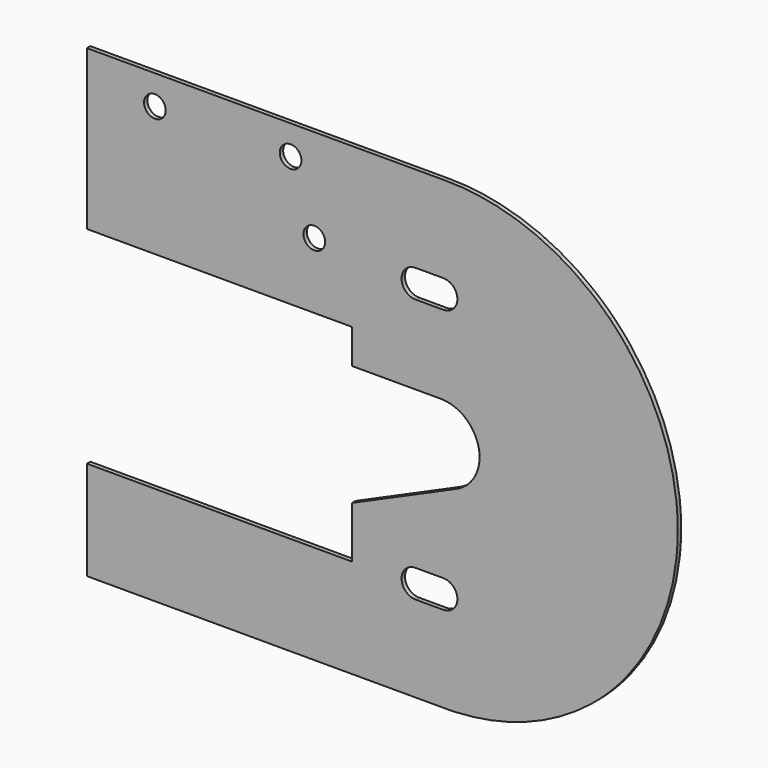
from build123d import *

# Parameters (mm, degrees)
F0_R     = 4.0005
F1_DEPTH = 1.5748


with BuildPart() as f1:
    # F0 (on Front) → F1 (new body)
    with BuildSketch(Plane.XZ):
        with BuildLine():
            Line((732.4313869209, 36.5125), (732.4313869209, 0))
            Line((732.4313869209, 0), (864.6383869209, 0))
            ThreePointArc((864.6383869209, 0), (866.7557920134, 0.0261539128), (868.8719051041, 0.1045996926))
            ThreePointArc((868.8719051041, 0.1045996926), (878.3590689291, 1.1051529768), (887.6763155537, 3.1536401389))
            ThreePointArc((887.6763155537, 3.1536401389), (903.696677756, 9.4149381337), (918.1445842563, 18.748418483))
            ThreePointArc((918.1445842563, 18.748418483), (921.7883869209, 21.8293575429), (925.2551157381, 25.1082711828))
            Line((925.2551157381, 25.1082711828), (873.8802209099, 76.483166011))
            ThreePointArc((873.8802209099, 76.483166011), (871.5444569052, 74.2857554291), (868.7774235028, 72.664665394))
            Line((868.7774235028, 72.664665394), (830.2213869209, 55.5625))
            Line((830.2213869209, 55.5625), (830.2213869209, 36.5125))
            Line((830.2213869209, 36.5125), (747.6713869209, 36.5125))
            Line((747.6713869209, 36.5125), (732.4313869209, 36.5125))
        make_face()
        with BuildLine():
            ThreePointArc((853.6528869209, 31.8135), (848.5093869209, 36.957), (853.6528869209, 42.1005))
            Line((853.6528869209, 42.1005), (863.9398869209, 42.1005))
            ThreePointArc((863.9398869209, 42.1005), (867.57689065, 40.594003729), (869.0833869209, 36.957))
            ThreePointArc((869.0833869209, 36.957), (867.57689065, 33.319996271), (863.9398869209, 31.8135))
            Line((863.9398869209, 31.8135), (853.6528869209, 31.8135))
        make_face(mode=Mode.SUBTRACT)
        with BuildLine():
            Line((732.4313869209, 112.7125), (747.6713869209, 112.7125))
            Line((747.6713869209, 112.7125), (830.2213869209, 112.7125))
            Line((830.2213869209, 112.7125), (830.2213869209, 100.0125))
            Line((830.2213869209, 100.0125), (862.984296866, 100.0125))
            ThreePointArc((862.984296866, 100.0125), (868.9880437433, 98.6898632728), (873.8802209099, 94.966833989))
            Line((873.8802209099, 94.966833989), (925.2551157381, 146.3417288172))
            ThreePointArc((925.2551157381, 146.3417288172), (921.7883869209, 149.6206424571), (918.1445842563, 152.701581517))
            ThreePointArc((918.1445842563, 152.701581517), (901.799905044, 162.9765190517), (883.5704291304, 169.3333333333))
            ThreePointArc((883.5704291304, 169.3333333333), (874.1633869209, 170.9191899427), (864.6383869209, 171.45))
            Line((864.6383869209, 171.45), (858.2883869209, 171.45))
            Line((858.2883869209, 171.45), (839.2383869209, 171.45))
            Line((839.2383869209, 171.45), (749.5336282768, 171.45))
            Line((749.5336282768, 171.45), (732.4313869209, 171.45))
            Line((732.4313869209, 171.45), (732.4313869209, 112.7125))
        make_face()
        with Locations((816.3148869209, 137.033)):
            Circle(F0_R, mode=Mode.SUBTRACT)
        with BuildLine():
            ThreePointArc((853.6528869209, 129.2225), (848.5093869209, 134.366), (853.6528869209, 139.5095))
            Line((853.6528869209, 139.5095), (863.9398869209, 139.5095))
            ThreePointArc((863.9398869209, 139.5095), (867.57689065, 138.003003729), (869.0833869209, 134.366))
            ThreePointArc((869.0833869209, 134.366), (867.57689065, 130.728996271), (863.9398869209, 129.2225))
            Line((863.9398869209, 129.2225), (853.6528869209, 129.2225))
        make_face(mode=Mode.SUBTRACT)
        with Locations((757.5138869209, 160.655)):
            Circle(F0_R, mode=Mode.SUBTRACT)
        with Locations((807.5772869209, 160.655)):
            Circle(F0_R, mode=Mode.SUBTRACT)
        with BuildLine():
            Line((873.8802209099, 76.483166011), (925.2551157381, 25.1082711828))
            ThreePointArc((925.2551157381, 25.1082711828), (928.534029378, 28.575), (931.6149684379, 32.2188026646))
            ThreePointArc((931.6149684379, 32.2188026646), (943.8379598455, 52.9194627605), (949.8325768637, 76.2))
            ThreePointArc((949.8325768637, 76.2), (950.2305815354, 80.9551104752), (950.3633869209, 85.725))
            Line((950.3633869209, 85.725), (877.271796866, 85.725))
            ThreePointArc((877.271796866, 85.725), (876.3971297328, 80.8027473921), (873.8802209099, 76.483166011))
        make_face()
        with BuildLine():
            ThreePointArc((873.8802209099, 94.966833989), (876.3971297328, 90.6472526079), (877.271796866, 85.725))
            Line((877.271796866, 85.725), (950.3633869209, 85.725))
            ThreePointArc((950.3633869209, 85.725), (950.2305815354, 90.4948895248), (949.8325768637, 95.25))
            ThreePointArc((949.8325768637, 95.25), (943.8379598455, 118.5305372395), (931.6149684379, 139.2311973354))
            ThreePointArc((931.6149684379, 139.2311973354), (928.534029378, 142.875), (925.2551157381, 146.3417288172))
            Line((925.2551157381, 146.3417288172), (873.8802209099, 94.966833989))
        make_face()
    extrude(amount=F1_DEPTH)


solid = f1.part
